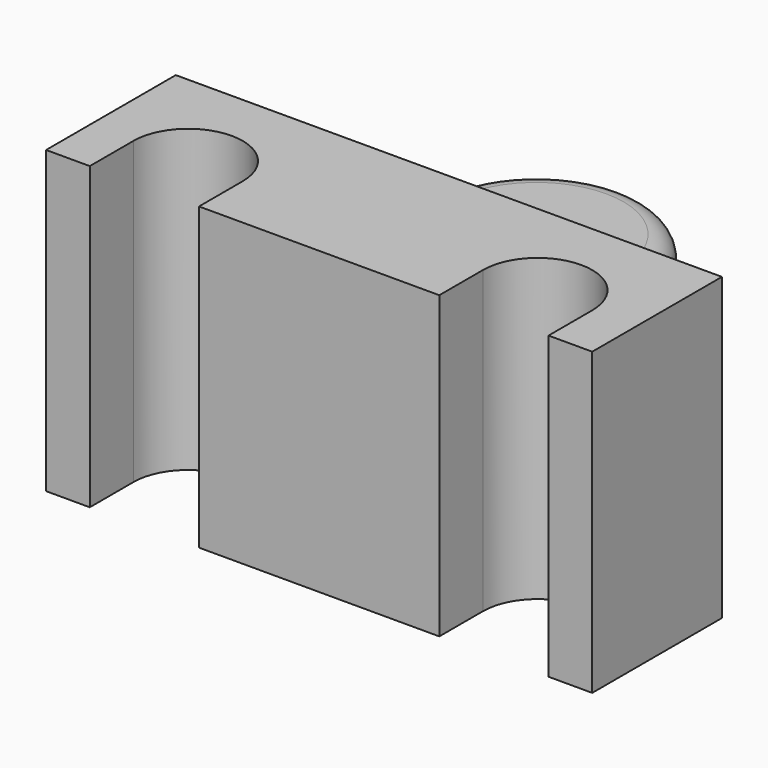
from build123d import *

# Parameters (mm, degrees)
F1_DEPTH     = 13.75
F2_W         = 10
F2_H         = 5
F3_DEPTH     = 10
F4_R         = 1
F5_T1_DEPTH  = 5
F5_T4_ANGLE  = 90
F5_T6_ANGLE  = 90
F5_T8_ANGLE  = 90
F5_T10_ANGLE = 90


# Not quite as in the source:
# - a fillet or chamfer that OpenCascade refuses, or shapes differently, is made with other operations: its cross-section is extruded or revolved along the edge and cut away or added


with BuildPart() as f1:
    # F0 (on Top) → F1 (new body)
    with BuildSketch(Plane.XY):
        with BuildLine():
            Line((7.9270144597, -2.8950429987), (-17.0730578044, -2.8950429987))
            Line((-17.0730578044, -2.8950429987), (-17.0730578044, -7.8164328754))
            Line((-17.0730578044, -7.8164328754), (-17.0730578044, -10.3164328754))
            Line((-17.0730578044, -10.3164328754), (-15.0730578044, -10.3164328754))
            Line((-15.0730578044, -10.3164328754), (-15.0730578044, -7.8164328754))
            ThreePointArc((-15.0730578044, -7.8164328754), (-12.5730578044, -5.3164328754), (-10.0730578044, -7.8164328754))
            Line((-10.0730578044, -7.8164328754), (-10.0730578044, -10.3164328754))
            Line((-10.0730578044, -10.3164328754), (0.9269421956, -10.3164328754))
            Line((0.9269421956, -10.3164328754), (0.9269421956, -7.8164328754))
            ThreePointArc((0.9269421956, -7.8164328754), (3.4269421956, -5.3164328754), (5.9269421956, -7.8164328754))
            Line((5.9269421956, -7.8164328754), (5.9269421956, -10.3164328754))
            Line((5.9269421956, -10.3164328754), (7.9270144597, -10.3164328754))
            Line((7.9270144597, -10.3164328754), (7.9270144597, -7.8164328754))
            Line((7.9270144597, -7.8164328754), (7.9270144597, -2.8950429987))
        make_face()
    extrude(amount=F1_DEPTH)

    # F2 (on face) → F3 (join)
    with BuildSketch(Plane(origin=(0, -2.8950429987, 0), x_dir=(-1, 0, 0), z_dir=(0, 1, 0))):
        with Locations((4.5730578044, 6.875)):
            Rectangle(F2_W, F2_H)
    extrude(amount=F3_DEPTH)

    # F4
    f4_edges = [f1.edges().sort_by_distance(p)[0] for p in [
        (-4.573058, 7.104957, 9.375),
        (-4.573058, 7.104957, 4.375),
        (-9.573058, 2.104957, 4.375),
        (-9.573058, 2.104957, 9.375),
        (0.426942, 2.104957, 9.375),
        (0.426942, 2.104957, 4.375),
    ]]
    fillet(f4_edges, radius=F4_R)

    # F5: fillet of radius 5 on 2 edges, made by hand

    # F5_s2 → F5_t1 (cut)
    with BuildSketch(Plane.XY.offset(4.375)):
        with BuildLine():
            ThreePointArc((-9.5730578044, 2.1049570013), (-8.1085917103, 5.6404909072), (-4.5730578044, 7.1049570013))
            Line((-4.5730578044, 7.1049570013), (-9.5730578044, 7.1049570013))
            Line((-9.5730578044, 7.1049570013), (-9.5730578044, 2.1049570013))
        make_face()
        with BuildLine():
            ThreePointArc((0.4269421956, 2.1049570013), (-1.0375238985, 5.6404909072), (-4.5730578044, 7.1049570013))
            Line((-4.5730578044, 7.1049570013), (0.4269421956, 7.1049570013))
            Line((0.4269421956, 7.1049570013), (0.4269421956, 2.1049570013))
        make_face()
    extrude(amount=F5_T1_DEPTH, mode=Mode.SUBTRACT)

    # F5_s3 → F5_t4 (revolve, cut)
    with BuildSketch(Plane.XZ.offset(-2.1049570013)):
        with BuildLine():
            ThreePointArc((-0.5730578044, 9.375), (0.1340489768, 9.0821067812), (0.4269421956, 8.375))
            Line((0.4269421956, 8.375), (0.4269421956, 9.375))
            Line((0.4269421956, 9.375), (-0.5730578044, 9.375))
        make_face()
    revolve(axis=Axis((-4.5730578044, 2.1049570013, 9.375), (0, 0, 1)), revolution_arc=F5_T4_ANGLE, mode=Mode.SUBTRACT)

    # F5_s5 → F5_t6 (revolve, cut)
    with BuildSketch(Plane.YZ.offset(-4.5730578044)):
        with BuildLine():
            ThreePointArc((6.1049570013, 4.375), (6.8120637825, 4.6678932188), (7.1049570013, 5.375))
            Line((7.1049570013, 5.375), (7.1049570013, 4.375))
            Line((7.1049570013, 4.375), (6.1049570013, 4.375))
        make_face()
    revolve(axis=Axis((-4.5730578044, 2.1049570013, 4.375), (0, 0, -1)), revolution_arc=F5_T6_ANGLE, mode=Mode.SUBTRACT)

    # F5_s7 → F5_t8 (revolve, cut)
    with BuildSketch(Plane.XZ.offset(-2.1049570013)):
        with BuildLine():
            ThreePointArc((-8.5730578044, 4.375), (-9.2801645856, 4.6678932188), (-9.5730578044, 5.375))
            Line((-9.5730578044, 5.375), (-9.5730578044, 4.375))
            Line((-9.5730578044, 4.375), (-8.5730578044, 4.375))
        make_face()
    revolve(axis=Axis((-4.5730578044, 2.1049570013, 4.375), (0, 0, -1)), revolution_arc=F5_T8_ANGLE, mode=Mode.SUBTRACT)

    # F5_s9 → F5_t10 (revolve, cut)
    with BuildSketch(Plane.YZ.offset(-4.5730578044)):
        with BuildLine():
            ThreePointArc((6.1049570013, 9.375), (6.8120637825, 9.0821067812), (7.1049570013, 8.375))
            Line((7.1049570013, 8.375), (7.1049570013, 9.375))
            Line((7.1049570013, 9.375), (6.1049570013, 9.375))
        make_face()
    revolve(axis=Axis((-4.5730578044, 2.1049570013, 9.375), (0, 0, 1)), revolution_arc=F5_T10_ANGLE, mode=Mode.SUBTRACT)


solid = f1.part
